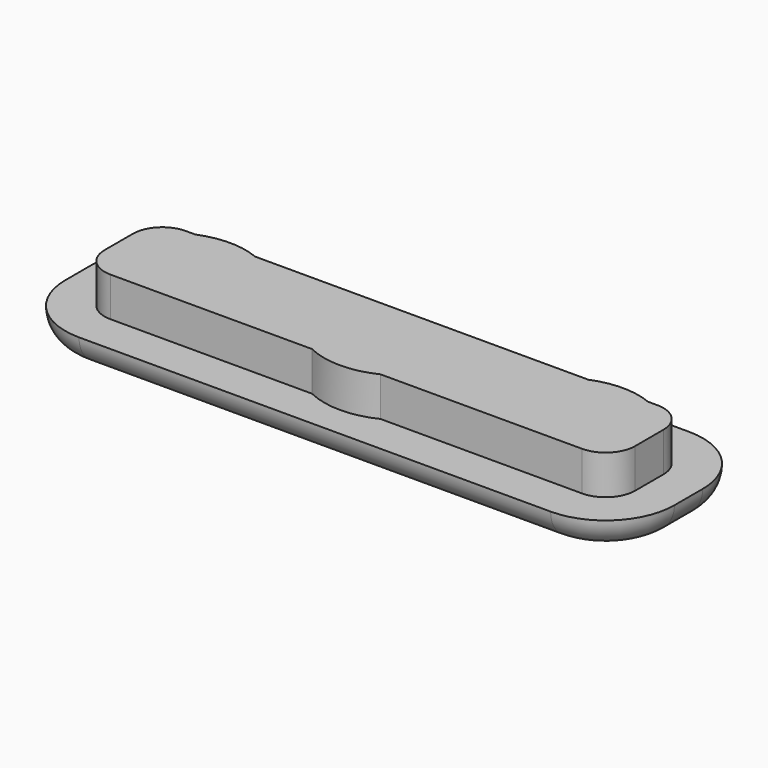
from build123d import *

# Parameters (mm, degrees)
F1_DEPTH = 1.5
F2_DEPTH = 3.5
F3_R     = 1.49999
F5_DEPTH = 2


# Not quite as in the source:
# - a fillet or chamfer is up to 0.001 mm smaller than in the source, because OpenCascade refuses the exact size


with BuildPart() as f1:
    # F0 (on Top) → F1 (new body)
    with BuildSketch(Plane.XY):
        with BuildLine():
            Line((15.5, -0.9), (15.5, 0.9))
            ThreePointArc((15.5, 0.9), (14.4748737342, 3.3748737342), (12, 4.4))
            Line((12, 4.4), (-12, 4.4))
            ThreePointArc((-12, 4.4), (-14.4748737342, 3.3748737342), (-15.5, 0.9))
            Line((-15.5, 0.9), (-15.5, -0.9))
            ThreePointArc((-15.5, -0.9), (-14.4748737342, -3.3748737342), (-12, -4.4))
            Line((-12, -4.4), (12, -4.4))
            ThreePointArc((12, -4.4), (14.4748737342, -3.3748737342), (15.5, -0.9))
        make_face()
        with BuildLine():
            ThreePointArc((13.5, -0.9), (13.0606601718, -1.9606601718), (12, -2.4))
            Line((12, -2.4), (-12, -2.4))
            ThreePointArc((-12, -2.4), (-13.0606601718, -1.9606601718), (-13.5, -0.9))
            Line((-13.5, -0.9), (-13.5, 0.9))
            ThreePointArc((-13.5, 0.9), (-13.0606601718, 1.9606601718), (-12, 2.4))
            Line((-12, 2.4), (12, 2.4))
            ThreePointArc((12, 2.4), (13.0606601718, 1.9606601718), (13.5, 0.9))
            Line((13.5, 0.9), (13.5, -0.9))
        make_face(mode=Mode.SUBTRACT)
        with BuildLine():
            Line((-12, -2.4), (12, -2.4))
            ThreePointArc((12, -2.4), (13.0606601718, -1.9606601718), (13.5, -0.9))
            Line((13.5, -0.9), (13.5, 0.9))
            ThreePointArc((13.5, 0.9), (13.0606601718, 1.9606601718), (12, 2.4))
            Line((12, 2.4), (-12, 2.4))
            ThreePointArc((-12, 2.4), (-13.0606601718, 1.9606601718), (-13.5, 0.9))
            Line((-13.5, 0.9), (-13.5, -0.9))
            ThreePointArc((-13.5, -0.9), (-13.0606601718, -1.9606601718), (-12, -2.4))
        make_face()
        with BuildLine():
            ThreePointArc((12, 1.6), (12.4949747468, 1.3949747468), (12.7, 0.9))
            Line((12.7, 0.9), (12.7, -0.9))
            ThreePointArc((12.7, -0.9), (12.4949747468, -1.3949747468), (12, -1.6))
            Line((12, -1.6), (-12, -1.6))
            ThreePointArc((-12, -1.6), (-12.4949747468, -1.3949747468), (-12.7, -0.9))
            Line((-12.7, -0.9), (-12.7, 0.9))
            ThreePointArc((-12.7, 0.9), (-12.4949747468, 1.3949747468), (-12, 1.6))
            Line((-12, 1.6), (12, 1.6))
        make_face(mode=Mode.SUBTRACT)
        with BuildLine():
            Line((12.7, -0.9), (12.7, 0.9))
            ThreePointArc((12.7, 0.9), (12.4949747468, 1.3949747468), (12, 1.6))
            Line((12, 1.6), (-12, 1.6))
            ThreePointArc((-12, 1.6), (-12.4949747468, 1.3949747468), (-12.7, 0.9))
            Line((-12.7, 0.9), (-12.7, -0.9))
            ThreePointArc((-12.7, -0.9), (-12.4949747468, -1.3949747468), (-12, -1.6))
            Line((-12, -1.6), (12, -1.6))
            ThreePointArc((12, -1.6), (12.4949747468, -1.3949747468), (12.7, -0.9))
        make_face()
    extrude(amount=F1_DEPTH)

    # F0 (on Top) → F2 (join)
    with BuildSketch(Plane.XY):
        with BuildLine():
            Line((-12, -2.4), (12, -2.4))
            ThreePointArc((12, -2.4), (13.0606601718, -1.9606601718), (13.5, -0.9))
            Line((13.5, -0.9), (13.5, 0.9))
            ThreePointArc((13.5, 0.9), (13.0606601718, 1.9606601718), (12, 2.4))
            Line((12, 2.4), (-12, 2.4))
            ThreePointArc((-12, 2.4), (-13.0606601718, 1.9606601718), (-13.5, 0.9))
            Line((-13.5, 0.9), (-13.5, -0.9))
            ThreePointArc((-13.5, -0.9), (-13.0606601718, -1.9606601718), (-12, -2.4))
        make_face()
        with BuildLine():
            ThreePointArc((12, 1.6), (12.4949747468, 1.3949747468), (12.7, 0.9))
            Line((12.7, 0.9), (12.7, -0.9))
            ThreePointArc((12.7, -0.9), (12.4949747468, -1.3949747468), (12, -1.6))
            Line((12, -1.6), (-12, -1.6))
            ThreePointArc((-12, -1.6), (-12.4949747468, -1.3949747468), (-12.7, -0.9))
            Line((-12.7, -0.9), (-12.7, 0.9))
            ThreePointArc((-12.7, 0.9), (-12.4949747468, 1.3949747468), (-12, 1.6))
            Line((-12, 1.6), (12, 1.6))
        make_face(mode=Mode.SUBTRACT)
        with BuildLine():
            Line((12.7, -0.9), (12.7, 0.9))
            ThreePointArc((12.7, 0.9), (12.4949747468, 1.3949747468), (12, 1.6))
            Line((12, 1.6), (-12, 1.6))
            ThreePointArc((-12, 1.6), (-12.4949747468, 1.3949747468), (-12.7, 0.9))
            Line((-12.7, 0.9), (-12.7, -0.9))
            ThreePointArc((-12.7, -0.9), (-12.4949747468, -1.3949747468), (-12, -1.6))
            Line((-12, -1.6), (12, -1.6))
            ThreePointArc((12, -1.6), (12.4949747468, -1.3949747468), (12.7, -0.9))
        make_face()
    extrude(amount=F2_DEPTH)

    # F3 (radius 1.5 in the source; OpenCascade refuses exactly that, so slightly less here)
    f3_edges = [f1.edges().sort_by_distance(p)[0] for p in [
        (0, -4.4, 0),
        (-14.474874, -3.374874, 0),
        (-15.5, 0, 0),
        (14.474874, -3.374874, 0),
        (15.5, 0, 0),
        (14.474874, 3.374874, 0),
        (0, 4.4, 0),
        (-14.474874, 3.374874, 0),
    ]]
    fillet(f3_edges, radius=F3_R)

    # F4 (on face) → F5 (join, through all)
    with BuildSketch(Plane.XY.offset(3.5)):
        with BuildLine():
            ThreePointArc((-6.1542230954, -2.4), (-6.0387434053, -1.8553793215), (-6, -1.3))
            ThreePointArc((-6, -1.3), (-6.6773900574, 0.9271648276), (-8.4801315846, 2.4))
            Line((-8.4801315846, 2.4), (-11.5198684154, 2.4))
            ThreePointArc((-11.5198684154, 2.4), (-12.6603120365, 1.6870955573), (-13.5, 0.6364916731))
            Line((-13.5, 0.6364916731), (-13.5, -0.9))
            ThreePointArc((-13.5, -0.9), (-13.0606601718, -1.9606601718), (-12, -2.4))
            Line((-12, -2.4), (-6.1542230954, -2.4))
        make_face()
        with BuildLine():
            Line((-11.5198684154, 2.4), (-8.4801315846, 2.4))
            ThreePointArc((-8.4801315846, 2.4), (-10, 2.7), (-11.5198684154, 2.4))
        make_face()
        with BuildLine():
            Line((3.8157568057, 2.4), (-3.8157568057, 2.4))
            ThreePointArc((-3.8157568057, 2.4), (-3.6723969913, -0.3854022638), (-1.7435595774, -2.4))
            Line((-1.7435595774, -2.4), (1.7435595774, -2.4))
            ThreePointArc((1.7435595774, -2.4), (3.3892652825, -0.9243542184), (4, 1.2))
            ThreePointArc((4, 1.2), (3.9536709033, 1.8070307971), (3.8157568057, 2.4))
        make_face()
        with BuildLine():
            Line((1.7435595774, -2.4), (-1.7435595774, -2.4))
            ThreePointArc((-1.7435595774, -2.4), (0, -2.8), (1.7435595774, -2.4))
        make_face()
        with BuildLine():
            ThreePointArc((11.5198684154, 2.4), (10, 2.7), (8.4801315846, 2.4))
            Line((8.4801315846, 2.4), (11.5198684154, 2.4))
        make_face()
    extrude(amount=-F5_DEPTH)


solid = f1.part
